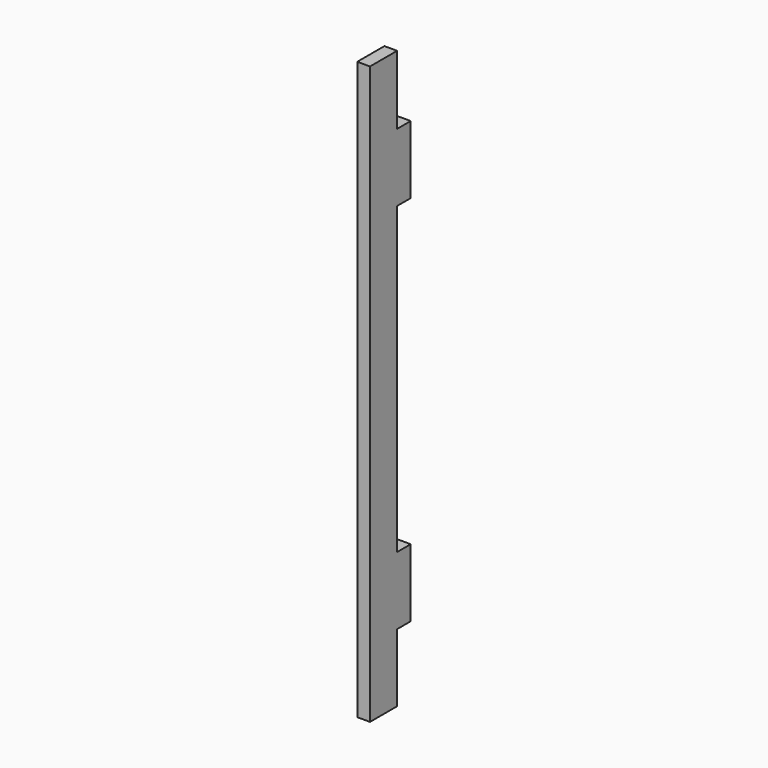
from build123d import *

# Parameters (mm, degrees)
F1_DEPTH = 19.05


# Not quite as in the source:
# - a length typed as a fraction of an inch, garbled in the dataset ("3 / 203.2 mm" for 3/8 in), is restored


with BuildPart() as f1:
    # F0 (on Right) → F1 (new body)
    with BuildSketch(Plane.YZ):
        Polygon((-24.5588049293, 447.4677373628), (-75.3588049293, 447.4677373628), (-75.3588049293, -416.1322626372), (-24.5588049293, -416.1322626372), (-24.5588049293, -314.5322626372), (0.8411950707, -314.5322626372), (0.8411950707, -212.9322626372), (-24.5588049293, -212.9322626372), (-24.5588049293, 243.0214576224), (0.8411950707, 243.0214576224), (0.8411950707, 344.6214576224), (-24.5588049293, 344.6214576224), align=None)
    extrude(amount=F1_DEPTH)


solid = f1.part
